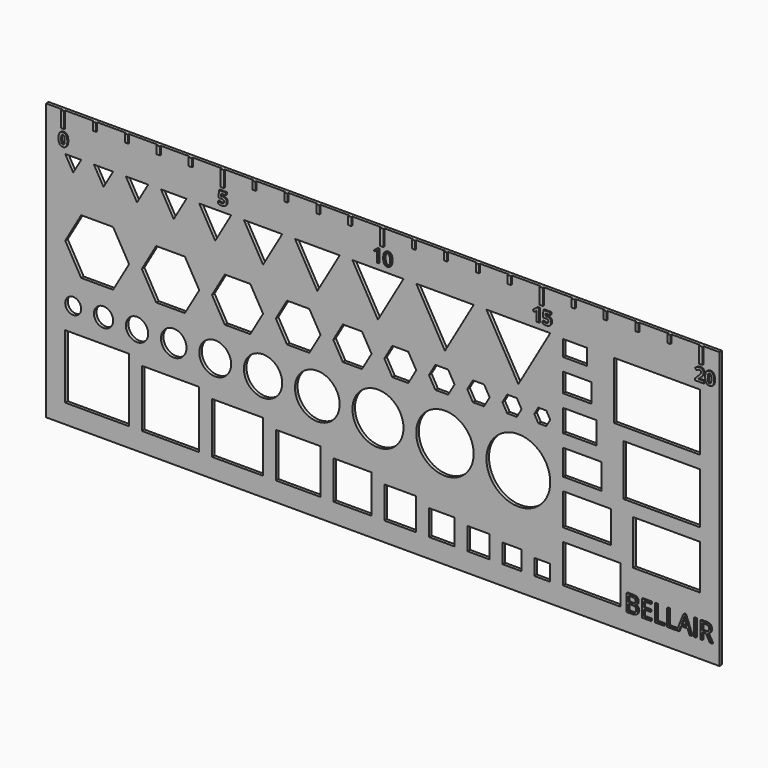
from build123d import *

# Parameters (mm, degrees)
F0_W         = 211
F0_H         = 86.6147367097
F0_W_2       = 20
F0_H_2       = 20
F0_W_3       = 18
F0_H_3       = 18
F0_W_4       = 16
F0_H_4       = 16
F0_W_5       = 14
F0_H_5       = 14
F0_W_6       = 12
F0_H_6       = 12
F0_R         = 2.5
F0_R_2       = 3
F0_R_3       = 3.5
F0_R_4       = 4
F0_R_5       = 5
F0_R_6       = 6
F0_R_7       = 7
F0_R_8       = 8
F0_W_7       = 8
F0_H_7       = 8
F0_W_8       = 7
F0_H_8       = 7
F0_W_9       = 6
F0_H_9       = 6
F0_W_10      = 5
F0_H_10      = 5
F0_W_11      = 10
F0_H_11      = 10
F0_R_9       = 9
F0_R_10      = 10
F0_W_12      = 15
F0_W_13      = 21
F0_W_14      = 10.5
F0_W_15      = 24
F0_W_16      = 9
F0_W_17      = 7.5
F0_W_18      = 27
F1_DEPTH     = 1
F2_TEXT_SIZE = 7.3304426082
F3_DEPTH     = 0.4
F5_W         = 1
F5_H         = 5
F5_H_2       = 2.5
F6_DEPTH     = 0.4


# Not quite as in the source:
# - Text() gives the source's letters only with a copy of the font that has no kerning and outlines rounded to 1/6400 em; it was checked with that copy


with BuildPart() as f1:
    # F0 (on Front) → F1 (new body)
    with BuildSketch(Plane.XZ):
        with Locations((99.5, 37.3073683549)):
            Rectangle(F0_W, F0_H)
        with Locations((10, 10)):
            Rectangle(F0_W_2, F0_H_2, mode=Mode.SUBTRACT)
        with Locations((33, 9)):
            Rectangle(F0_W_3, F0_H_3, mode=Mode.SUBTRACT)
        with Locations((54, 8)):
            Rectangle(F0_W_4, F0_H_4, mode=Mode.SUBTRACT)
        with Locations((73, 7)):
            Rectangle(F0_W_5, F0_H_5, mode=Mode.SUBTRACT)
        with Locations((90, 6)):
            Rectangle(F0_W_6, F0_H_6, mode=Mode.SUBTRACT)
        with Locations((2.5, 27.5)):
            Circle(F0_R, mode=Mode.SUBTRACT)
        with Locations((12, 27.5)):
            Circle(F0_R_2, mode=Mode.SUBTRACT)
        with Locations((22.5, 27.5)):
            Circle(F0_R_3, mode=Mode.SUBTRACT)
        with Locations((34, 27.5)):
            Circle(F0_R_4, mode=Mode.SUBTRACT)
        with Locations((47, 27.5)):
            Circle(F0_R_5, mode=Mode.SUBTRACT)
        with Locations((62, 27.5)):
            Circle(F0_R_6, mode=Mode.SUBTRACT)
        with Locations((79, 27.5)):
            Circle(F0_R_7, mode=Mode.SUBTRACT)
        with Locations((98, 27.5)):
            Circle(F0_R_8, mode=Mode.SUBTRACT)
        with Locations((118, 4)):
            Rectangle(F0_W_7, F0_H_7, mode=Mode.SUBTRACT)
        with Locations((129.5, 3.5)):
            Rectangle(F0_W_8, F0_H_8, mode=Mode.SUBTRACT)
        with Locations((140, 3)):
            Rectangle(F0_W_9, F0_H_9, mode=Mode.SUBTRACT)
        with Locations((149.5, 2.5)):
            Rectangle(F0_W_10, F0_H_10, mode=Mode.SUBTRACT)
        with Locations((105, 5)):
            Rectangle(F0_W_11, F0_H_11, mode=Mode.SUBTRACT)
        with Locations((165, 6.3147367097)):
            Rectangle(F0_W_3, F0_H_6, mode=Mode.SUBTRACT)
        with Locations((119, 27.5)):
            Circle(F0_R_9, mode=Mode.SUBTRACT)
        with Locations((142, 27.5)):
            Circle(F0_R_10, mode=Mode.SUBTRACT)
        with Locations((163.5, 21.3147367097)):
            Rectangle(F0_W_12, F0_H_11, mode=Mode.SUBTRACT)
        with Locations((188.5, 19.3147367097)):
            Rectangle(F0_W_13, F0_H_5, mode=Mode.SUBTRACT)
        with Locations((162, 34.3147367097)):
            Rectangle(F0_W_6, F0_H_7, mode=Mode.SUBTRACT)
        Polygon((0, 44.6961524227), (5, 53.3564064606), (15, 53.3564064606), (20, 44.6961524227), (15, 36.0358983849), (5, 36.0358983849), align=None, mode=Mode.SUBTRACT)
        Polygon((42, 44.6961524227), (37.5, 36.9019237886), (28.5, 36.9019237886), (24, 44.6961524227), (28.5, 52.4903810568), (37.5, 52.4903810568), align=None, mode=Mode.SUBTRACT)
        Polygon((46, 44.6961524227), (50, 51.624355653), (58, 51.624355653), (62, 44.6961524227), (58, 37.7679491924), (50, 37.7679491924), align=None, mode=Mode.SUBTRACT)
        Polygon((66, 44.6961524227), (69.5, 50.7583302492), (76.5, 50.7583302492), (80, 44.6961524227), (76.5, 38.6339745962), (69.5, 38.6339745962), align=None, mode=Mode.SUBTRACT)
        Polygon((84, 44.6961524227), (87, 49.8923048454), (93, 49.8923048454), (96, 44.6961524227), (93, 39.5), (87, 39.5), align=None, mode=Mode.SUBTRACT)
        Polygon((2.5, 64.2846096908), (0, 68.6147367097), (5, 68.6147367097), align=None, mode=Mode.SUBTRACT)
        Polygon((12, 63.418584287), (9, 68.6147367097), (15, 68.6147367097), align=None, mode=Mode.SUBTRACT)
        Polygon((22.5, 62.5525588833), (19, 68.6147367097), (26, 68.6147367097), align=None, mode=Mode.SUBTRACT)
        Polygon((34, 61.6865334795), (30, 68.6147367097), (38, 68.6147367097), align=None, mode=Mode.SUBTRACT)
        Polygon((47, 59.9544826719), (42, 68.6147367097), (52, 68.6147367097), align=None, mode=Mode.SUBTRACT)
        Polygon((62, 58.2224318643), (56, 68.6147367097), (68, 68.6147367097), align=None, mode=Mode.SUBTRACT)
        Polygon((79, 56.4903810568), (72, 68.6147367097), (86, 68.6147367097), align=None, mode=Mode.SUBTRACT)
        Polygon((98, 54.7583302492), (90, 68.6147367097), (106, 68.6147367097), align=None, mode=Mode.SUBTRACT)
        Polygon((100, 44.6961524227), (102.5, 49.0262794416), (107.5, 49.0262794416), (110, 44.6961524227), (107.5, 40.3660254038), (102.5, 40.3660254038), align=None, mode=Mode.SUBTRACT)
        Polygon((114, 44.6961524227), (116, 48.1602540378), (120, 48.1602540378), (122, 44.6961524227), (120, 41.2320508076), (116, 41.2320508076), align=None, mode=Mode.SUBTRACT)
        Polygon((126, 44.6961524227), (127.75, 47.727241336), (131.25, 47.727241336), (133, 44.6961524227), (131.25, 41.6650635095), (127.75, 41.6650635095), align=None, mode=Mode.SUBTRACT)
        Polygon((137, 44.6961524227), (138.5, 47.2942286341), (141.5, 47.2942286341), (143, 44.6961524227), (141.5, 42.0980762114), (138.5, 42.0980762114), align=None, mode=Mode.SUBTRACT)
        Polygon((147, 44.6961524227), (148.25, 46.8612159322), (150.75, 46.8612159322), (152, 44.6961524227), (150.75, 42.5310889132), (148.25, 42.5310889132), align=None, mode=Mode.SUBTRACT)
        with Locations((161.25, 45.8147367097)):
            Rectangle(F0_W_14, F0_H_8, mode=Mode.SUBTRACT)
        with Locations((187, 38.3147367097)):
            Rectangle(F0_W_15, F0_H_4, mode=Mode.SUBTRACT)
        with Locations((160.5, 56.3147367097)):
            Rectangle(F0_W_16, F0_H_9, mode=Mode.SUBTRACT)
        Polygon((119, 53.0262794416), (110, 68.6147367097), (128, 68.6147367097), align=None, mode=Mode.SUBTRACT)
        Polygon((142, 51.2942286341), (132, 68.6147367097), (152, 68.6147367097), align=None, mode=Mode.SUBTRACT)
        with Locations((159.75, 65.8147367097)):
            Rectangle(F0_W_17, F0_H_10, mode=Mode.SUBTRACT)
        with Locations((185.5, 59.3147367097)):
            Rectangle(F0_W_18, F0_H_3, mode=Mode.SUBTRACT)
    extrude(amount=F1_DEPTH)

    # F2 (on face) → F3 (join)
    with BuildSketch(Plane.XZ.offset(1)):
        with Locations((175.5508746406, -0.2779186779)):
            Text('BELLAIR', F2_TEXT_SIZE, font='Open Sans', text_align=(TextAlign.LEFT, TextAlign.BOTTOM))
    extrude(amount=F3_DEPTH)

    # F5 (on face) → F6 (join)
    with BuildSketch(Plane.XZ.offset(1)):
        with Locations((-0.5, 78.1147367097)):
            Rectangle(F5_W, F5_H)
        with Locations((9.5, 79.3647367097)):
            Rectangle(F5_W, F5_H_2)
        with Locations((19.5, 79.3647367097)):
            Rectangle(F5_W, F5_H_2)
        with Locations((29.5, 79.3647367097)):
            Rectangle(F5_W, F5_H_2)
        with Locations((39.5, 79.3647367097)):
            Rectangle(F5_W, F5_H_2)
        with Locations((49.5, 78.1147367097)):
            Rectangle(F5_W, F5_H)
        with Locations((59.5, 79.3647367097)):
            Rectangle(F5_W, F5_H_2)
        with Locations((69.5, 79.3647367097)):
            Rectangle(F5_W, F5_H_2)
        with Locations((79.5, 79.3647367097)):
            Rectangle(F5_W, F5_H_2)
        with Locations((89.5, 79.3647367097)):
            Rectangle(F5_W, F5_H_2)
        with Locations((99.5, 78.1147367097)):
            Rectangle(F5_W, F5_H)
        with Locations((109.5, 79.3647367097)):
            Rectangle(F5_W, F5_H_2)
        with Locations((119.5, 79.3647367097)):
            Rectangle(F5_W, F5_H_2)
        with Locations((129.5, 79.3647367097)):
            Rectangle(F5_W, F5_H_2)
        with Locations((139.5, 79.3647367097)):
            Rectangle(F5_W, F5_H_2)
        with Locations((149.5, 78.1147367097)):
            Rectangle(F5_W, F5_H)
        with Locations((159.5, 79.3647367097)):
            Rectangle(F5_W, F5_H_2)
        with Locations((169.5, 79.3647367097)):
            Rectangle(F5_W, F5_H_2)
        with Locations((179.5, 79.3647367097)):
            Rectangle(F5_W, F5_H_2)
        with Locations((189.5, 79.3647367097)):
            Rectangle(F5_W, F5_H_2)
        with Locations((199.5, 78.1147367097)):
            Rectangle(F5_W, F5_H)
        with BuildLine():
            Line((98, 73.4411255986), (98, 70.6147367097))
            Line((98, 70.6147367097), (98.4392361111, 70.6147367097))
            Line((98.4392361111, 70.6147367097), (98.4392361111, 74.5808825431))
            Line((98.4392361111, 74.5808825431), (98.0598958333, 74.5808825431))
            Line((98.0598958333, 74.5808825431), (97.0104166667, 73.7692505986))
            Line((97.0104166667, 73.7692505986), (97.2491319444, 73.4602228209))
            add(Edge.make_bspline(
                [(97.89453125, 73.989302682), (97.8237847222, 73.9272367097), (97.2491319444, 73.4602228209)],
                knots=[0, 0, 0, 1, 1, 1], degree=2))
            add(Edge.make_bspline(
                [(98.0217013889, 74.1086603209), (97.9652777778, 74.0513686542), (97.89453125, 73.989302682)],
                knots=[0, 0, 0, 1, 1, 1], degree=2))
            add(Edge.make_bspline(
                [(98, 73.4411255986), (98, 73.7944242097), (98.0217013889, 74.1086603209)],
                knots=[0, 0, 0, 1, 1, 1], degree=2))
        make_face()
        with BuildLine():
            add(Edge.make_bspline(
                [(0.0126322815, 70.6147367097), (-0.1814376392, 70.5600492097), (-0.4157986111, 70.5600492097)],
                knots=[0.6691374514, 0.6691374514, 0.6691374514, 1, 1, 1], degree=2))
            Line((0.0126322815, 70.6147367097), (-0.8271688379, 70.6147367097))
            add(Edge.make_bspline(
                [(-0.4157986111, 70.5600492097), (-0.639413675, 70.5600492097), (-0.8271688379, 70.6147367097)],
                knots=[0, 0, 0, 0.3256694736, 0.3256694736, 0.3256694736], degree=2))
        make_face()
        with BuildLine():
            Line((-0.8271688379, 70.6147367097), (0.0126322815, 70.6147367097))
            add(Edge.make_bspline(
                [(0.6328125, 71.059615182), (0.405119895, 70.7253368805), (0.0126322815, 70.6147367097)],
                knots=[0, 0, 0, 0.6691374514, 0.6691374514, 0.6691374514], degree=2))
            add(Edge.make_bspline(
                [(0.9730902778, 72.5973755986), (0.9730902778, 71.5591811542), (0.6328125, 71.059615182)],
                knots=[0, 0, 0, 1, 1, 1], degree=2))
            add(Edge.make_bspline(
                [(0.6219618056, 74.1225492097), (0.9730902778, 73.6017158764), (0.9730902778, 72.5973755986)],
                knots=[0, 0, 0, 1, 1, 1], degree=2))
            add(Edge.make_bspline(
                [(-0.4157986111, 74.6433825431), (0.2708333333, 74.6433825431), (0.6219618056, 74.1225492097)],
                knots=[0, 0, 0, 1, 1, 1], degree=2))
            add(Edge.make_bspline(
                [(-1.4600694444, 74.145552682), (-1.1206597222, 74.6433825431), (-0.4157986111, 74.6433825431)],
                knots=[0, 0, 0, 1, 1, 1], degree=2))
            add(Edge.make_bspline(
                [(-1.7994791667, 72.5973755986), (-1.7994791667, 73.6477228209), (-1.4600694444, 74.145552682)],
                knots=[0, 0, 0, 1, 1, 1], degree=2))
            add(Edge.make_bspline(
                [(-1.4509548611, 71.0756742097), (-1.7994791667, 71.5912992097), (-1.7994791667, 72.5973755986)],
                knots=[0, 0, 0, 1, 1, 1], degree=2))
            add(Edge.make_bspline(
                [(-0.8271688379, 70.6147367097), (-1.2159342827, 70.7279725321), (-1.4509548611, 71.0756742097)],
                knots=[0.3256694736, 0.3256694736, 0.3256694736, 1, 1, 1], degree=2))
        make_face()
        with BuildLine():
            add(Edge.make_bspline(
                [(-0.9661458333, 72.5973755986), (-0.9661458333, 71.868208932), (-0.8402777778, 71.5522367097)],
                knots=[0, 0, 0, 1, 1, 1], degree=2))
            add(Edge.make_bspline(
                [(-0.8389756944, 73.6459867097), (-0.9661458333, 73.3274103209), (-0.9661458333, 72.5973755986)],
                knots=[0, 0, 0, 1, 1, 1], degree=2))
            add(Edge.make_bspline(
                [(-0.4157986111, 73.9645630986), (-0.7118055556, 73.9645630986), (-0.8389756944, 73.6459867097)],
                knots=[0, 0, 0, 1, 1, 1], degree=2))
            add(Edge.make_bspline(
                [(0.0060763889, 73.6459867097), (-0.1258680556, 73.9645630986), (-0.4157986111, 73.9645630986)],
                knots=[0, 0, 0, 1, 1, 1], degree=2))
            add(Edge.make_bspline(
                [(0.1380208333, 72.5973755986), (0.1380208333, 73.3274103209), (0.0060763889, 73.6459867097)],
                knots=[0, 0, 0, 1, 1, 1], degree=2))
            add(Edge.make_bspline(
                [(0.0078125, 71.5561429597), (0.1380208333, 71.876021432), (0.1380208333, 72.5973755986)],
                knots=[0, 0, 0, 1, 1, 1], degree=2))
            add(Edge.make_bspline(
                [(-0.4157986111, 71.2362644875), (-0.1223958333, 71.2362644875), (0.0078125, 71.5561429597)],
                knots=[0, 0, 0, 1, 1, 1], degree=2))
            add(Edge.make_bspline(
                [(-0.8402777778, 71.5522367097), (-0.7144097222, 71.2362644875), (-0.4157986111, 71.2362644875)],
                knots=[0, 0, 0, 1, 1, 1], degree=2))
        make_face(mode=Mode.SUBTRACT)
        with BuildLine():
            add(Edge.make_bspline(
                [(49.8818602254, 70.6147367097), (49.6379492982, 70.5600492097), (49.3402777778, 70.5600492097)],
                knots=[0.6094332671, 0.6094332671, 0.6094332671, 1, 1, 1], degree=2))
            Line((49.8818602254, 70.6147367097), (48.7365962974, 70.6147367097))
            add(Edge.make_bspline(
                [(49.3402777778, 70.5600492097), (49.0057795224, 70.5600492097), (48.7365962974, 70.6147367097)],
                knots=[0, 0, 0, 0.5050353738, 0.5050353738, 0.5050353738], degree=2))
        make_face()
        with BuildLine():
            Line((48.7365962974, 70.6147367097), (49.8818602254, 70.6147367097))
            add(Edge.make_bspline(
                [(50.5121527778, 70.9185561542), (50.2624544253, 70.7000700958), (49.8818602254, 70.6147367097)],
                knots=[0, 0, 0, 0.6094332671, 0.6094332671, 0.6094332671], degree=2))
            add(Edge.make_bspline(
                [(50.921875, 71.9411255986), (50.921875, 71.2770630986), (50.5121527778, 70.9185561542)],
                knots=[0, 0, 0, 1, 1, 1], degree=2))
            add(Edge.make_bspline(
                [(50.5811631944, 72.8256742097), (50.921875, 72.5027575431), (50.921875, 71.9411255986)],
                knots=[0, 0, 0, 1, 1, 1], degree=2))
            add(Edge.make_bspline(
                [(49.6657986111, 73.1485908764), (50.2404513889, 73.1485908764), (50.5811631944, 72.8256742097)],
                knots=[0, 0, 0, 1, 1, 1], degree=2))
            add(Edge.make_bspline(
                [(49.2560763889, 73.110396432), (49.421875, 73.1485908764), (49.6657986111, 73.1485908764)],
                knots=[0, 0, 0, 1, 1, 1], degree=2))
            Line((49.2560763889, 73.110396432), (49.1614583333, 73.0912992097))
            Line((49.1614583333, 73.0912992097), (49.234375, 73.8699450431))
            Line((49.234375, 73.8699450431), (50.6501736111, 73.8699450431))
            Line((50.6501736111, 73.8699450431), (50.6501736111, 74.5808825431))
            Line((50.6501736111, 74.5808825431), (48.4991319444, 74.5808825431))
            Line((48.4991319444, 74.5808825431), (48.3498263889, 72.5600492097))
            Line((48.3498263889, 72.5600492097), (48.6840277778, 72.3803617097))
            add(Edge.make_bspline(
                [(48.9661458333, 72.4419936542), (48.7925347222, 72.4133478209), (48.6840277778, 72.3803617097)],
                knots=[0, 0, 0, 1, 1, 1], degree=2))
            add(Edge.make_bspline(
                [(49.2829861111, 72.4706394875), (49.1397569444, 72.4706394875), (48.9661458333, 72.4419936542)],
                knots=[0, 0, 0, 1, 1, 1], degree=2))
            add(Edge.make_bspline(
                [(50.078125, 71.8708130986), (50.078125, 72.4706394875), (49.2829861111, 72.4706394875)],
                knots=[0, 0, 0, 1, 1, 1], degree=2))
            add(Edge.make_bspline(
                [(49.3098958333, 71.2414728209), (50.078125, 71.2414728209), (50.078125, 71.8708130986)],
                knots=[0, 0, 0, 1, 1, 1], degree=2))
            add(Edge.make_bspline(
                [(48.7703993056, 71.313521432), (49.0555555556, 71.2414728209), (49.3098958333, 71.2414728209)],
                knots=[0, 0, 0, 1, 1, 1], degree=2))
            add(Edge.make_bspline(
                [(48.2717013889, 71.4992853209), (48.4852430556, 71.3855700431), (48.7703993056, 71.313521432)],
                knots=[0, 0, 0, 1, 1, 1], degree=2))
            Line((48.2717013889, 71.4992853209), (48.2717013889, 70.774458932))
            add(Edge.make_bspline(
                [(48.7365962974, 70.6147367097), (48.4727807683, 70.6683337039), (48.2717013889, 70.774458932)],
                knots=[0.5050353738, 0.5050353738, 0.5050353738, 1, 1, 1], degree=2))
        make_face()
        with BuildLine():
            add(Edge.make_bspline(
                [(201.8438381066, 70.6147367097), (201.4550726617, 70.7279725321), (201.2200520833, 71.0756742097)],
                knots=[0.3256694736, 0.3256694736, 0.3256694736, 1, 1, 1], degree=2))
            Line((201.8438381066, 70.6147367097), (202.6836392259, 70.6147367097))
            add(Edge.make_bspline(
                [(203.3038194444, 71.059615182), (203.0761268395, 70.7253368805), (202.6836392259, 70.6147367097)],
                knots=[0, 0, 0, 0.6691374514, 0.6691374514, 0.6691374514], degree=2))
            add(Edge.make_bspline(
                [(203.6440972222, 72.5973755986), (203.6440972222, 71.5591811542), (203.3038194444, 71.059615182)],
                knots=[0, 0, 0, 1, 1, 1], degree=2))
            add(Edge.make_bspline(
                [(203.29296875, 74.1225492097), (203.6440972222, 73.6017158764), (203.6440972222, 72.5973755986)],
                knots=[0, 0, 0, 1, 1, 1], degree=2))
            add(Edge.make_bspline(
                [(202.2552083333, 74.6433825431), (202.9418402778, 74.6433825431), (203.29296875, 74.1225492097)],
                knots=[0, 0, 0, 1, 1, 1], degree=2))
            add(Edge.make_bspline(
                [(201.2109375, 74.145552682), (201.5503472222, 74.6433825431), (202.2552083333, 74.6433825431)],
                knots=[0, 0, 0, 1, 1, 1], degree=2))
            add(Edge.make_bspline(
                [(200.8715277778, 72.5973755986), (200.8715277778, 73.6477228209), (201.2109375, 74.145552682)],
                knots=[0, 0, 0, 1, 1, 1], degree=2))
            add(Edge.make_bspline(
                [(201.2200520833, 71.0756742097), (200.8715277778, 71.5912992097), (200.8715277778, 72.5973755986)],
                knots=[0, 0, 0, 1, 1, 1], degree=2))
        make_face()
        with BuildLine():
            add(Edge.make_bspline(
                [(201.7048611111, 72.5973755986), (201.7048611111, 71.868208932), (201.8307291667, 71.5522367097)],
                knots=[0, 0, 0, 1, 1, 1], degree=2))
            add(Edge.make_bspline(
                [(201.83203125, 73.6459867097), (201.7048611111, 73.3274103209), (201.7048611111, 72.5973755986)],
                knots=[0, 0, 0, 1, 1, 1], degree=2))
            add(Edge.make_bspline(
                [(202.2552083333, 73.9645630986), (201.9592013889, 73.9645630986), (201.83203125, 73.6459867097)],
                knots=[0, 0, 0, 1, 1, 1], degree=2))
            add(Edge.make_bspline(
                [(202.6770833333, 73.6459867097), (202.5451388889, 73.9645630986), (202.2552083333, 73.9645630986)],
                knots=[0, 0, 0, 1, 1, 1], degree=2))
            add(Edge.make_bspline(
                [(202.8090277778, 72.5973755986), (202.8090277778, 73.3274103209), (202.6770833333, 73.6459867097)],
                knots=[0, 0, 0, 1, 1, 1], degree=2))
            add(Edge.make_bspline(
                [(202.6788194444, 71.5561429597), (202.8090277778, 71.876021432), (202.8090277778, 72.5973755986)],
                knots=[0, 0, 0, 1, 1, 1], degree=2))
            add(Edge.make_bspline(
                [(202.2552083333, 71.2362644875), (202.5486111111, 71.2362644875), (202.6788194444, 71.5561429597)],
                knots=[0, 0, 0, 1, 1, 1], degree=2))
            add(Edge.make_bspline(
                [(201.8307291667, 71.5522367097), (201.9565972222, 71.2362644875), (202.2552083333, 71.2362644875)],
                knots=[0, 0, 0, 1, 1, 1], degree=2))
        make_face(mode=Mode.SUBTRACT)
        with BuildLine():
            Line((202.6836392259, 70.6147367097), (201.8438381066, 70.6147367097))
            add(Edge.make_bspline(
                [(202.2552083333, 70.5600492097), (202.0315932694, 70.5600492097), (201.8438381066, 70.6147367097)],
                knots=[0, 0, 0, 0.3256694736, 0.3256694736, 0.3256694736], degree=2))
            add(Edge.make_bspline(
                [(202.6836392259, 70.6147367097), (202.4895693053, 70.5600492097), (202.2552083333, 70.5600492097)],
                knots=[0.6691374514, 0.6691374514, 0.6691374514, 1, 1, 1], degree=2))
        make_face()
        with BuildLine():
            Line((197.7222222222, 71.1980700431), (197.7222222222, 70.6147367097))
            Line((197.7222222222, 70.6147367097), (200.4947916667, 70.6147367097))
            Line((200.4947916667, 70.6147367097), (200.4947916667, 71.3204658764))
            Line((200.4947916667, 71.3204658764), (198.7664930556, 71.3204658764))
            Line((198.7664930556, 71.3204658764), (198.7664930556, 71.3577922653))
            Line((198.7664930556, 71.3577922653), (199.2769097222, 71.8378269875))
            add(Edge.make_bspline(
                [(199.9887152778, 72.5570110153), (199.7864583333, 72.3048408764), (199.2769097222, 71.8378269875)],
                knots=[0, 0, 0, 1, 1, 1], degree=2))
            add(Edge.make_bspline(
                [(200.2873263889, 73.0491985153), (200.1909722222, 72.8091811542), (199.9887152778, 72.5570110153)],
                knots=[0, 0, 0, 1, 1, 1], degree=2))
            add(Edge.make_bspline(
                [(200.3836805556, 73.563521432), (200.3836805556, 73.2892158764), (200.2873263889, 73.0491985153)],
                knots=[0, 0, 0, 1, 1, 1], degree=2))
            add(Edge.make_bspline(
                [(200.2261284722, 74.122115182), (200.3836805556, 73.8777575431), (200.3836805556, 73.563521432)],
                knots=[0, 0, 0, 1, 1, 1], degree=2))
            add(Edge.make_bspline(
                [(199.7838541667, 74.5018894875), (200.0685763889, 74.3664728209), (200.2261284722, 74.122115182)],
                knots=[0, 0, 0, 1, 1, 1], degree=2))
            add(Edge.make_bspline(
                [(199.1276041667, 74.6373061542), (199.4991319444, 74.6373061542), (199.7838541667, 74.5018894875)],
                knots=[0, 0, 0, 1, 1, 1], degree=2))
            add(Edge.make_bspline(
                [(198.6176215278, 74.5817505986), (198.8454861111, 74.6373061542), (199.1276041667, 74.6373061542)],
                knots=[0, 0, 0, 1, 1, 1], degree=2))
            add(Edge.make_bspline(
                [(198.1970486111, 74.4233304597), (198.3897569444, 74.5261950431), (198.6176215278, 74.5817505986)],
                knots=[0, 0, 0, 1, 1, 1], degree=2))
            add(Edge.make_bspline(
                [(197.7118055556, 74.0704658764), (198.0043402778, 74.3204658764), (198.1970486111, 74.4233304597)],
                knots=[0, 0, 0, 1, 1, 1], degree=2))
            Line((197.7118055556, 74.0704658764), (198.1675347222, 73.5305353209))
            add(Edge.make_bspline(
                [(198.6206597222, 73.8317505986), (198.4036458333, 73.7258478209), (198.1675347222, 73.5305353209)],
                knots=[0, 0, 0, 1, 1, 1], degree=2))
            add(Edge.make_bspline(
                [(199.0677083333, 73.9376533764), (198.8376736111, 73.9376533764), (198.6206597222, 73.8317505986)],
                knots=[0, 0, 0, 1, 1, 1], degree=2))
            add(Edge.make_bspline(
                [(199.4192708333, 73.8208999042), (199.2873263889, 73.9376533764), (199.0677083333, 73.9376533764)],
                knots=[0, 0, 0, 1, 1, 1], degree=2))
            add(Edge.make_bspline(
                [(199.5512152778, 73.4654311542), (199.5512152778, 73.704146432), (199.4192708333, 73.8208999042)],
                knots=[0, 0, 0, 1, 1, 1], degree=2))
            add(Edge.make_bspline(
                [(199.4913194444, 73.1564033764), (199.5512152778, 73.305708932), (199.5512152778, 73.4654311542)],
                knots=[0, 0, 0, 1, 1, 1], degree=2))
            add(Edge.make_bspline(
                [(199.2960069444, 72.8321846264), (199.4314236111, 73.0070978209), (199.4913194444, 73.1564033764)],
                knots=[0, 0, 0, 1, 1, 1], degree=2))
            add(Edge.make_bspline(
                [(198.7178819444, 72.204146432), (199.1605902778, 72.657271432), (199.2960069444, 72.8321846264)],
                knots=[0, 0, 0, 1, 1, 1], degree=2))
            Line((198.7178819444, 72.204146432), (197.7222222222, 71.1980700431))
        make_face()
        with BuildLine():
            add(Edge.make_bspline(
                [(150.4076032419, 70.6147367097), (150.1437877127, 70.6683337039), (149.9427083333, 70.774458932)],
                knots=[0.5050353738, 0.5050353738, 0.5050353738, 1, 1, 1], degree=2))
            Line((150.4076032419, 70.6147367097), (151.5528671698, 70.6147367097))
            add(Edge.make_bspline(
                [(152.1831597222, 70.9185561542), (151.9334613697, 70.7000700958), (151.5528671698, 70.6147367097)],
                knots=[0, 0, 0, 0.6094332671, 0.6094332671, 0.6094332671], degree=2))
            add(Edge.make_bspline(
                [(152.5928819444, 71.9411255986), (152.5928819444, 71.2770630986), (152.1831597222, 70.9185561542)],
                knots=[0, 0, 0, 1, 1, 1], degree=2))
            add(Edge.make_bspline(
                [(152.2521701389, 72.8256742097), (152.5928819444, 72.5027575431), (152.5928819444, 71.9411255986)],
                knots=[0, 0, 0, 1, 1, 1], degree=2))
            add(Edge.make_bspline(
                [(151.3368055556, 73.1485908764), (151.9114583333, 73.1485908764), (152.2521701389, 72.8256742097)],
                knots=[0, 0, 0, 1, 1, 1], degree=2))
            add(Edge.make_bspline(
                [(150.9270833333, 73.110396432), (151.0928819444, 73.1485908764), (151.3368055556, 73.1485908764)],
                knots=[0, 0, 0, 1, 1, 1], degree=2))
            Line((150.9270833333, 73.110396432), (150.8324652778, 73.0912992097))
            Line((150.8324652778, 73.0912992097), (150.9053819444, 73.8699450431))
            Line((150.9053819444, 73.8699450431), (152.3211805556, 73.8699450431))
            Line((152.3211805556, 73.8699450431), (152.3211805556, 74.5808825431))
            Line((152.3211805556, 74.5808825431), (150.1701388889, 74.5808825431))
            Line((150.1701388889, 74.5808825431), (150.0208333333, 72.5600492097))
            Line((150.0208333333, 72.5600492097), (150.3550347222, 72.3803617097))
            add(Edge.make_bspline(
                [(150.6371527778, 72.4419936542), (150.4635416667, 72.4133478209), (150.3550347222, 72.3803617097)],
                knots=[0, 0, 0, 1, 1, 1], degree=2))
            add(Edge.make_bspline(
                [(150.9539930556, 72.4706394875), (150.8107638889, 72.4706394875), (150.6371527778, 72.4419936542)],
                knots=[0, 0, 0, 1, 1, 1], degree=2))
            add(Edge.make_bspline(
                [(151.7491319444, 71.8708130986), (151.7491319444, 72.4706394875), (150.9539930556, 72.4706394875)],
                knots=[0, 0, 0, 1, 1, 1], degree=2))
            add(Edge.make_bspline(
                [(150.9809027778, 71.2414728209), (151.7491319444, 71.2414728209), (151.7491319444, 71.8708130986)],
                knots=[0, 0, 0, 1, 1, 1], degree=2))
            add(Edge.make_bspline(
                [(150.44140625, 71.313521432), (150.7265625, 71.2414728209), (150.9809027778, 71.2414728209)],
                knots=[0, 0, 0, 1, 1, 1], degree=2))
            add(Edge.make_bspline(
                [(149.9427083333, 71.4992853209), (150.15625, 71.3855700431), (150.44140625, 71.313521432)],
                knots=[0, 0, 0, 1, 1, 1], degree=2))
            Line((149.9427083333, 71.4992853209), (149.9427083333, 70.774458932))
        make_face()
        with BuildLine():
            Line((151.5528671698, 70.6147367097), (150.4076032419, 70.6147367097))
            add(Edge.make_bspline(
                [(151.0112847222, 70.5600492097), (150.6767864669, 70.5600492097), (150.4076032419, 70.6147367097)],
                knots=[0, 0, 0, 0.5050353738, 0.5050353738, 0.5050353738], degree=2))
            add(Edge.make_bspline(
                [(151.5528671698, 70.6147367097), (151.3089562426, 70.5600492097), (151.0112847222, 70.5600492097)],
                knots=[0.6094332671, 0.6094332671, 0.6094332671, 1, 1, 1], degree=2))
        make_face()
        with BuildLine():
            Line((147.9565972222, 72.9098755986), (147.9565972222, 70.6147367097))
            Line((147.9565972222, 70.6147367097), (148.7951388889, 70.6147367097))
            Line((148.7951388889, 70.6147367097), (148.7951388889, 74.5808825431))
            Line((148.7951388889, 74.5808825431), (148.1059027778, 74.5808825431))
            Line((148.1059027778, 74.5808825431), (146.828125, 73.563521432))
            Line((146.828125, 73.563521432), (147.2326388889, 73.0591811542))
            Line((147.2326388889, 73.0591811542), (147.6883680556, 73.4255005986))
            add(Edge.make_bspline(
                [(147.9782986111, 73.6989380986), (147.7699652778, 73.4906047653), (147.6883680556, 73.4255005986)],
                knots=[0, 0, 0, 1, 1, 1], degree=2))
            Line((147.9782986111, 73.6989380986), (147.9652777778, 73.2866117097))
            Line((147.9652777778, 73.2866117097), (147.9565972222, 72.9098755986))
        make_face()
        with BuildLine():
            add(Edge.make_bspline(
                [(100.8774969737, 70.6147367097), (100.5123712909, 70.7286074051), (100.2868923611, 71.0795804597)],
                knots=[0.3244428423, 0.3244428423, 0.3244428423, 1, 1, 1], degree=2))
            Line((100.8774969737, 70.6147367097), (101.6617230487, 70.6147367097))
            add(Edge.make_bspline(
                [(102.2521701389, 71.067427682), (102.0343941531, 70.7266242985), (101.6617230487, 70.6147367097)],
                knots=[0, 0, 0, 0.6716946069, 0.6716946069, 0.6716946069], degree=2))
            add(Edge.make_bspline(
                [(102.5763888889, 72.6034519875), (102.5763888889, 71.5748061542), (102.2521701389, 71.067427682)],
                knots=[0, 0, 0, 1, 1, 1], degree=2))
            add(Edge.make_bspline(
                [(102.2413194444, 74.1195110153), (102.5763888889, 73.5956394875), (102.5763888889, 72.6034519875)],
                knots=[0, 0, 0, 1, 1, 1], degree=2))
            add(Edge.make_bspline(
                [(101.2604166667, 74.6433825431), (101.90625, 74.6433825431), (102.2413194444, 74.1195110153)],
                knots=[0, 0, 0, 1, 1, 1], degree=2))
            add(Edge.make_bspline(
                [(100.2760416667, 74.1412124042), (100.5989583333, 74.6433825431), (101.2604166667, 74.6433825431)],
                knots=[0, 0, 0, 1, 1, 1], degree=2))
            add(Edge.make_bspline(
                [(99.953125, 72.6034519875), (99.953125, 73.6390422653), (100.2760416667, 74.1412124042)],
                knots=[0, 0, 0, 1, 1, 1], degree=2))
            add(Edge.make_bspline(
                [(100.2868923611, 71.0795804597), (99.953125, 71.5991117097), (99.953125, 72.6034519875)],
                knots=[0, 0, 0, 1, 1, 1], degree=2))
        make_face()
        with BuildLine():
            add(Edge.make_bspline(
                [(100.4088541667, 72.6034519875), (100.4088541667, 71.7380005986), (100.6124131944, 71.3430353209)],
                knots=[0, 0, 0, 1, 1, 1], degree=2))
            add(Edge.make_bspline(
                [(100.6124131944, 73.8608304597), (100.4088541667, 73.4689033764), (100.4088541667, 72.6034519875)],
                knots=[0, 0, 0, 1, 1, 1], degree=2))
            add(Edge.make_bspline(
                [(101.2604166667, 74.2527575431), (100.8159722222, 74.2527575431), (100.6124131944, 73.8608304597)],
                knots=[0, 0, 0, 1, 1, 1], degree=2))
            add(Edge.make_bspline(
                [(101.9127604167, 73.8551880986), (101.7109375, 74.2527575431), (101.2604166667, 74.2527575431)],
                knots=[0, 0, 0, 1, 1, 1], degree=2))
            add(Edge.make_bspline(
                [(102.1145833333, 72.6034519875), (102.1145833333, 73.4576186542), (101.9127604167, 73.8551880986)],
                knots=[0, 0, 0, 1, 1, 1], degree=2))
            add(Edge.make_bspline(
                [(101.9127604167, 71.3482436542), (102.1145833333, 71.7484172653), (102.1145833333, 72.6034519875)],
                knots=[0, 0, 0, 1, 1, 1], degree=2))
            add(Edge.make_bspline(
                [(101.2604166667, 70.9480700431), (101.7109375, 70.9480700431), (101.9127604167, 71.3482436542)],
                knots=[0, 0, 0, 1, 1, 1], degree=2))
            add(Edge.make_bspline(
                [(100.6124131944, 71.3430353209), (100.8159722222, 70.9480700431), (101.2604166667, 70.9480700431)],
                knots=[0, 0, 0, 1, 1, 1], degree=2))
        make_face(mode=Mode.SUBTRACT)
        with BuildLine():
            Line((101.6617230487, 70.6147367097), (100.8774969737, 70.6147367097))
            add(Edge.make_bspline(
                [(101.2604166667, 70.5600492097), (101.0528521053, 70.5600492097), (100.8774969737, 70.6147367097)],
                knots=[0, 0, 0, 0.3244428423, 0.3244428423, 0.3244428423], degree=2))
            add(Edge.make_bspline(
                [(101.6617230487, 70.6147367097), (101.4795719161, 70.5600492097), (101.2604166667, 70.5600492097)],
                knots=[0.6716946069, 0.6716946069, 0.6716946069, 1, 1, 1], degree=2))
        make_face()
    extrude(amount=F6_DEPTH)


solid = f1.part
